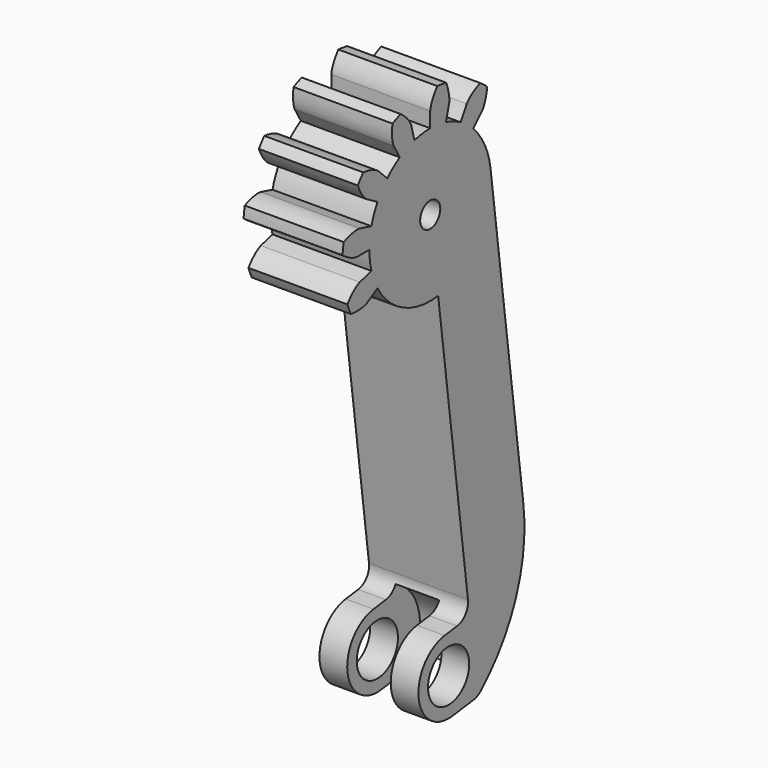
from build123d import *

# Parameters (mm, degrees)
F3_DEPTH        = 10
F3_COPIES_COUNT = 5
F3_COPIES_ANGLE = 120
F5_R            = 4.7625
F6_DEPTH        = 8
F7_R            = 1.27
F8_DEPTH        = 25.4
F10_DEPTH       = 25.4
F12_DEPTH       = 10
F15_DEPTH       = 2
F17_R           = 2.6
F18_DEPTH       = 10
F20_W           = 4.4
F20_H           = 5.3975


# Not quite as in the source:
# - a feature of the source that left no trace in its solid (it failed there, or was rolled back) is left out
# - a pattern or mirror of a feature is missing from the dataset's text; its kind, count and spacing are read off the source's solid
# - a feature names something its author has since deleted; it is built from what else it names


with BuildPart() as f3:
    # F2 (on Right) → F3 (new body)
    with BuildSketch(Plane.YZ):
        with BuildLine():
            ThreePointArc((-7.6882625, 0), (0, -7.6882625), (7.6882625, 0))
            ThreePointArc((7.6882625, 0), (1.0035196289, 7.6224883485), (-7.426291308, 1.9898687587))
            ThreePointArc((-7.426291308, 1.9898687587), (-7.6224883485, 1.0035196289), (-7.6882625, 0))
        make_face()
        with BuildLine():
            ThreePointArc((-7.6882625, 0), (-7.6224883485, 1.0035196289), (-7.426291308, 1.9898687587))
            Line((-7.426291308, 1.9898687587), (-8.9073876605, 2.3867273303))
            add(Edge.make_bspline(
                [(-8.9073876605, 2.3867273303), (-8.9129675505, 2.3882224573), (-8.9176841258, 2.3891504576), (-8.9560398208, 2.3967560952), (-9.0111204055, 2.4040860623), (-9.0921767557, 2.4112581523), (-9.1956464181, 2.4150161111), (-9.3225341112, 2.4133585936), (-9.4721001001, 2.4038885647), (-9.6439830376, 2.3843397936), (-9.8372804848, 2.3525439817), (-10.0518635466, 2.3059720142), (-10.2838045034, 2.2438455399), (-10.5435425365, 2.158650335), (-10.7314150502, 2.0892946498), (-10.888833847, 2.0216630994), (-10.9303977099, 2.003512454)],
                knots=[0, 0, 0, 0, 0.0202164122, 0.055231725, 0.1004362437, 0.1539229332, 0.2145711301, 0.2816202297, 0.3545102827, 0.4328067574, 0.5161597183, 0.6042794907, 0.6969211254, 0.7938739525, 0.8949542617, 0.934249932, 0.934249932, 0.934249932, 0.934249932], degree=3))
            ThreePointArc((-10.9303977099, 2.003512454), (-11.017431022, 1.450472311), (-11.0765006198, 0.8937506752))
            add(Edge.make_bspline(
                [(-9.2216062746, 0), (-9.2273830018, 0), (-9.2321790478, 0.0003243601), (-9.2711962881, 0.0029050627), (-9.3262971825, 0.0100807624), (-9.406447878, 0.0241319827), (-9.5073645284, 0.0472819925), (-9.6294996312, 0.081723983), (-9.7715182587, 0.1295818548), (-9.9324848329, 0.1929510955), (-10.1109664676, 0.273692552), (-10.3061840768, 0.3742158014), (-10.5141423223, 0.4942561043), (-10.742979855, 0.6437735028), (-10.9065001958, 0.7593909349), (-11.0410507439, 0.8654609788), (-11.0765006198, 0.8937506752)],
                knots=[0, 0, 0, 0, 0.0202164122, 0.055231725, 0.1004362437, 0.1539229332, 0.2145711301, 0.2816202297, 0.3545102827, 0.4328067574, 0.5161597183, 0.6042794907, 0.6969211254, 0.7938739525, 0.8949542617, 0.934249932, 0.934249932, 0.934249932, 0.934249932], degree=3))
            Line((-9.2216062746, 0), (-7.6882625, 0))
        make_face()
    extrude(amount=F3_DEPTH)

    # F3_copies: F3 ×5 about axis
    f3_copies_axis = Axis((0, 0, 0), (-1, 0, 0))


with BuildPart() as f3_1:
    add(f3.part)
    for i in range(1, F3_COPIES_COUNT):
        add(f3.part.rotate(f3_copies_axis, i * F3_COPIES_ANGLE / (F3_COPIES_COUNT - 1)))

    # F3_copies1: F3 across plane


with BuildPart() as f3_2:
    add(f3_1.part)
    add(f3_1.part.mirror(Plane(origin=(0, 0, 0), x_dir=(0, -0.9914448614, -0.1305261922), z_dir=(0, 0.1305261922, -0.9914448614))))

    # F5 (on face) → F6 (cut)
    with BuildSketch(Plane(origin=(0, 0, 0), x_dir=(0, -1, 0), z_dir=(-1, 0, 0))):
        Circle(F5_R)
    extrude(amount=-F6_DEPTH, mode=Mode.SUBTRACT)

    # F7 (on face) → F8 (cut)
    with BuildSketch(Plane.YZ.offset(10)):
        Circle(F7_R)
    extrude(amount=-F8_DEPTH, mode=Mode.SUBTRACT)

    # F9 (on face) → F10 (cut)
    with BuildSketch(Plane.YZ.offset(10)):
        with BuildLine():
            Line((5.4364225493, 5.4364225493), (6.4313569287, -2.1208543547))
            Line((6.4313569287, -2.1208543547), (-6.658230636, -3.84413125))
            ThreePointArc((-6.658230636, -3.84413125), (-1.0393271028, -17.0218990639), (10.0434558029, -7.9445886398))
            ThreePointArc((10.0434558029, -7.9445886398), (14.9426168475, 1.225772556), (5.4364225493, 5.4364225493))
        make_face()
    extrude(amount=-F10_DEPTH, mode=Mode.SUBTRACT)

    # F11 (on face) → F12 (join)
    with BuildSketch(Plane(origin=(0, 0, 0), x_dir=(0, -1, 0), z_dir=(-1, 0, 0))):
        with BuildLine():
            ThreePointArc((3.3289323807, -3.4058208195), (-0.6216309904, -4.7217561523), (-4.0969930528, -2.4281791893))
            Line((-4.0969930528, -2.4281791893), (-6.4313569287, -2.1208543547))
            Line((-6.4313569287, -2.1208543547), (-5.4364225493, 5.4364225493))
            ThreePointArc((-5.4364225493, 5.4364225493), (-6.895393066, 3.4004315512), (-7.6224883485, 1.0035196289))
            Line((-7.6224883485, 1.0035196289), (-8.6260079774, -6.6189687196))
            Line((-8.6260079774, -6.6189687196), (-1.0035196289, -7.6224883485))
            ThreePointArc((-1.0035196289, -7.6224883485), (3.4004315512, -6.895393066), (6.658230636, -3.84413125))
            Line((6.658230636, -3.84413125), (3.3289323807, -3.4058208195))
        make_face()
    extrude(amount=-F12_DEPTH)

    # F13: union 

    # F14 (on face) → F15 (join)
    with BuildSketch(Plane.YZ.offset(10)):
        with BuildLine():
            Line((4.0969930528, -2.4281791893), (-3.3289323807, -3.4058208195))
            ThreePointArc((-3.3289323807, -3.4058208195), (0.6216309904, -4.7217561523), (4.0969930528, -2.4281791893))
        make_face()
    extrude(amount=-F15_DEPTH)

    # F16: union 

    # F17 (on face) → F18 (join)
    with BuildSketch(Plane.YZ.offset(10)):
        with BuildLine():
            Line((11.7666949515, -30.4748547197), (8.6260079774, -6.6189687196))
            Line((8.6260079774, -6.6189687196), (1.0035196289, -7.6224883485))
            Line((1.0035196289, -7.6224883485), (4.7658375934, -36.2001305009))
            ThreePointArc((4.7658375934, -36.2001305009), (4.4513673037, -37.3737495996), (3.3991292062, -37.9812595485))
            Line((3.3991292062, -37.9812595485), (1.8252104887, -38.1884698786))
            ThreePointArc((1.8252104887, -38.1884698786), (-1.4548896408, -42.4631795928), (2.8198200734, -45.7432797223))
            Line((2.8198200734, -45.7432797223), (5.4986207311, -45.3906089252))
            ThreePointArc((5.4986207311, -45.3906089252), (5.9506497242, -45.2608369332), (6.3448233333, -45.0043254397))
            ThreePointArc((6.3448233333, -45.0043254397), (10.8646203429, -38.4145914885), (11.7666949515, -30.4748547197))
        make_face()
        with Locations((2.3225152811, -41.9658748005)):
            Circle(F17_R, mode=Mode.SUBTRACT)
    extrude(amount=-F18_DEPTH)

    # F20 (on face) → F21 (revolve, cut)
    with BuildSketch(Plane(origin=(0, -3.1478374349, -0.4144206603), x_dir=(-1, 0, 0), z_dir=(0, 0.9914448614, 0.1305261922))):
        with Locations((-5, -39.21125)):
            Rectangle(F20_W, F20_H)
    revolve(axis=Axis((5.7694689557, 2.3225152811, -41.9658748005), (1, 0, 0)), mode=Mode.SUBTRACT)


solid = f3_2.part
